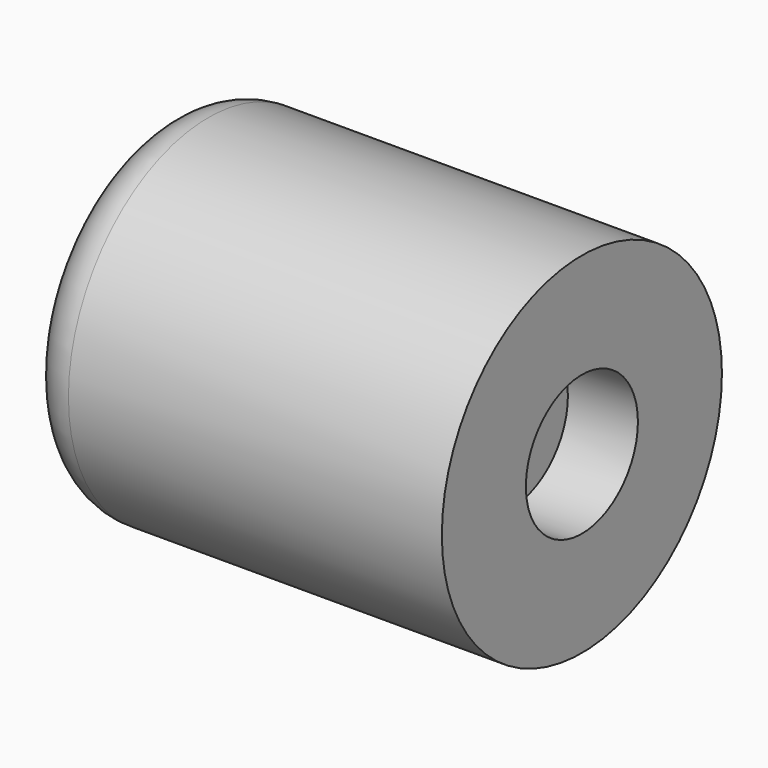
from build123d import *

# Parameters (mm, degrees)
F0_W      = 34
F0_H      = 24
F0_W_2    = 30
F0_H_2    = 20
F1_DEPTH  = 20
F2_R      = 6.5
F3_DEPTH  = 11.7
F4_R      = 7.5
F5_DEPTH  = 8.3
F6_R      = 7.5
F7_DEPTH  = 18
F8_R      = 2
F9_R      = 0.99999
F10_W     = 2
F10_H     = 20
F11_DEPTH = 25
F13_DEPTH = 15
F14_R     = 0.99999
F16_R     = 3
F17_DEPTH = 5
F18_W     = 40.3561908752
F18_H     = 35.6408245862
F20_DEPTH = 56.6
F21_DEPTH = 74.7


# Not quite as in the source:
# - a fillet or chamfer is up to 0.001 mm smaller than in the source, because OpenCascade refuses the exact size
# - a feature of the source that left no trace in its solid (it failed there, or was rolled back) is left out


with BuildPart() as f1:
    # F0 (on Front) → F1 (new body)
    with BuildSketch(Plane.XZ):
        Rectangle(F0_W, F0_H)
        Rectangle(F0_W_2, F0_H_2, mode=Mode.SUBTRACT)
    extrude(amount=F1_DEPTH)

    # F2 (on face) → F3 (cut)
    with BuildSketch(Plane.XY.offset(12)):
        with Locations((6, -10)):
            Circle(F2_R)
    extrude(amount=-F3_DEPTH, mode=Mode.SUBTRACT)

    # F4 (on face) → F5 (cut)
    with BuildSketch(Plane(origin=(0, 0, -12), x_dir=(1, 0, 0), z_dir=(0, 0, -1))):
        with Locations((-5, 10)):
            Circle(F4_R)
    extrude(amount=-F5_DEPTH, mode=Mode.SUBTRACT)

    # F6 (on face) → F7 (join)
    with BuildSketch(Plane(origin=(-17, 0, 0), x_dir=(0, -1, 0), z_dir=(-1, 0, 0))):
        with Locations((10, 0)):
            Circle(F6_R)
    extrude(amount=F7_DEPTH)

    # F8
    f8_edges = [f1.edges().sort_by_distance(p)[0] for p in [
        (-17, -10, 12),
        (-17, -10, -12),
        (-35, -2.5, 0),
    ]]
    fillet(f8_edges, radius=F8_R)

    # F9 (radius 1 in the source; OpenCascade refuses exactly that, so slightly less here)
    f9_edges = [f1.edges().sort_by_distance(p)[0] for p in [
        (-0.5, -10, 10),
        (-0.5, -10, 12),
        (-12.5, -10, -10),
        (-12.5, -10, -12),
    ]]
    fillet(f9_edges, radius=F9_R)

    # F10 (on face) → F11 (cut)
    with BuildSketch(Plane.XZ.offset(20)):
        with Locations((16, 0)):
            Rectangle(F10_W, F10_H)
    extrude(amount=-F11_DEPTH, mode=Mode.SUBTRACT)

    # F12 (on Right) → F13 (join, symmetric)
    with BuildSketch(Plane.YZ):
        with BuildLine():
            Line((-20, 10), (-20, 12))
            ThreePointArc((-20, 12), (-21, 11), (-20, 10))
        make_face()
        with BuildLine():
            Line((-19, 10), (-20, 10))
            ThreePointArc((-20, 10), (-19.5, 9.5), (-19, 10))
        make_face()
        with BuildLine():
            Line((-20, -12), (-20, -10))
            ThreePointArc((-20, -10), (-21, -11), (-20, -12))
        make_face()
        with BuildLine():
            Line((-19, -12), (-20, -12))
            ThreePointArc((-20, -12), (-19.5, -12.5), (-19, -12))
        make_face()
        with BuildLine():
            Line((0, -10), (0, -12))
            ThreePointArc((0, -12), (1, -11), (0, -10))
        make_face()
        with BuildLine():
            ThreePointArc((-1, -12), (-0.5, -12.5), (0, -12))
            Line((0, -12), (-1, -12))
        make_face()
        with BuildLine():
            Line((0, 12), (0, 10))
            ThreePointArc((0, 10), (1, 11), (0, 12))
        make_face()
        with BuildLine():
            ThreePointArc((-1, 10), (-0.5, 9.5), (0, 10))
            Line((0, 10), (-1, 10))
        make_face()
    extrude(amount=F13_DEPTH, both=True)

    # F14 (radius 1 in the source; OpenCascade refuses exactly that, so slightly less here)
    f14_edges = [f1.edges().sort_by_distance(p)[0] for p in [
        (15, -21, 11),
        (-15, -21, 11),
        (-15, -21, -11),
        (15, -21, -11),
        (-15, 1, 11),
        (-15, 1, -11),
        (15, 1, -11),
        (15, 1, 11),
    ]]
    fillet(f14_edges, radius=F14_R)

    # F16 (on face) → F17 (cut)
    with BuildSketch(Plane.YZ.offset(-15)):
        with Locations((-10, 0)):
            Circle(F16_R)
    extrude(amount=-F17_DEPTH, mode=Mode.SUBTRACT)


with BuildPart() as f19_1:
    # F19: copy of F1
    add(f1.part)


with BuildPart() as f20_tool:
    # F18 (on face) → F20 (new body)
    with BuildSketch(Plane(origin=(-17, 0, 0), x_dir=(0, -1, 0), z_dir=(-1, 0, 0))):
        with Locations((8.2543967292, -4.1322950274)):
            Rectangle(F18_W, F18_H)
    extrude(amount=-F20_DEPTH)


with BuildPart() as f1_1:
    add(f1.part)

    # F20: cut by f20_tool
    add(f20_tool.part, mode=Mode.SUBTRACT)

    # F18 (on face) → F21 (cut)
    with BuildSketch(Plane(origin=(-17, 0, 0), x_dir=(0, -1, 0), z_dir=(-1, 0, 0))):
        with Locations((8.2543967292, -4.1322950274)):
            Rectangle(F18_W, F18_H)
    extrude(amount=-F21_DEPTH, mode=Mode.SUBTRACT)


with BuildPart() as f19_1_1:
    add(f19_1.part)

    # F20: cut by f20_tool
    add(f20_tool.part, mode=Mode.SUBTRACT)


solid = Compound([f1_1.part, f19_1_1.part])
